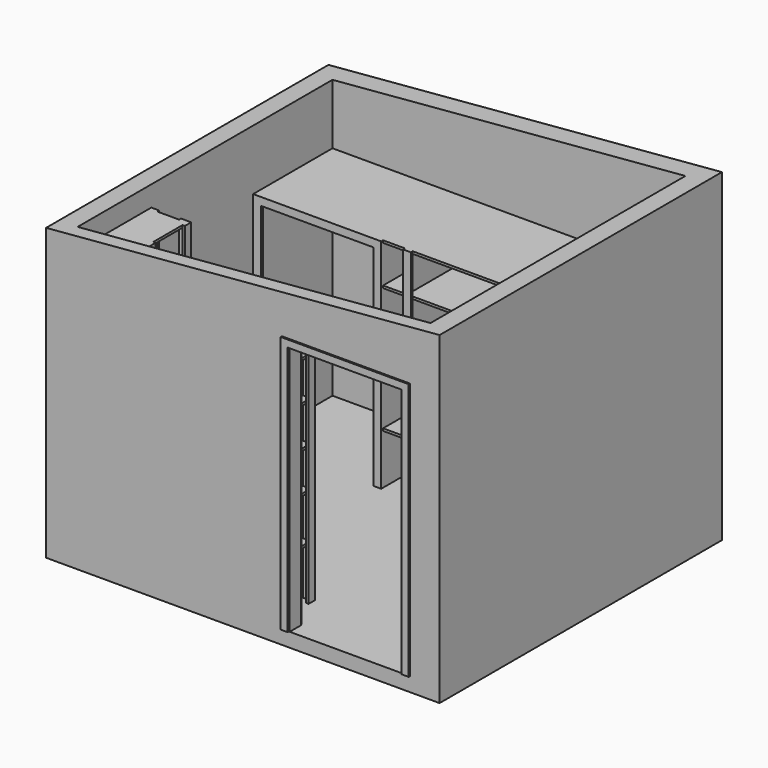
from build123d import *

# Parameters (mm, degrees)
F0_W      = 2590.8
F0_H      = 2520.95
F1_DEPTH  = 165.1
F2_W      = 3035.3
F2_H      = 2520.95
F3_DEPTH  = 114.3
F4_W      = 3035.3
F4_H      = 2520.95
F5_DEPTH  = 165.1
F6_W      = 2870.2
F6_H      = 2520.95
F7_DEPTH  = 165.1
F10_DEPTH = 2870.201
F8_W      = 914.4
F8_H      = 2032
F11_DEPTH = 114.3
F12_W     = 3200.4
F12_H     = 2870.2
F13_DEPTH = 114.3
F15_DEPTH = 12.7
F18_W     = 1651
F18_H     = 19.05
F19_DEPTH = 304.8
F20_W     = 1651
F20_H     = 38.1
F21_DEPTH = 19.05
F22_W     = 19.05
F22_H     = 63.5
F22_W_2   = 63.5
F22_H_2   = 19.05
F23_DEPTH = 2095.5
F24_W     = 2286
F24_H     = 19.05
F25_DEPTH = 304.8
F26_W     = 1422.4
F26_H     = 787.4
F26_W_2   = 990.6
F27_DEPTH = 990.6
F28_W     = 19.05
F28_H     = 787.4
F28_W_2   = 63.5
F28_H_2   = 19.05
F29_DEPTH = 1447.8
F30_W     = 19.05
F30_H     = 787.4
F31_DEPTH = 19.05
F32_W     = 2565.4
F32_H     = 787.4
F33_DEPTH = 19.05
F34_W     = 1631.95
F34_H     = 19.05
F35_DEPTH = 787.4
F36_W     = 1219.2
F36_H     = 2266.95
F37_DEPTH = 2520.951
F38_W     = 63.5
F38_H     = 19.05
F38_W_2   = 19.05
F38_H_2   = 787.4
F39_DEPTH = 1771.65
F40_W     = 19.05
F40_H     = 787.4
F41_DEPTH = 19.05
F42_W     = 2870.2
F42_H     = 787.4
F43_DEPTH = 19.05
F44_W     = 19.05
F44_H     = 323.85
F45_DEPTH = 787.4
F46_W     = 63.5
F46_H     = 19.05
F47_DEPTH = 323.85
F48_W     = 177.8
F48_H     = 19.05
F49_DEPTH = 787.4
F50_W     = 406.4
F50_H     = 19.05
F51_DEPTH = 304.8
F52_W     = 19.05
F52_H     = 63.5
F52_W_2   = 63.5
F52_H_2   = 19.05
F53_DEPTH = 2095.5
F54_W     = 914.4
F54_H     = 44.45
F54_H_2   = 19.05
F55_DEPTH = 19.05


# Not quite as in the source:
# - a pattern or mirror of a feature is missing from the dataset's text; its kind, count and spacing are read off the source's solid


with BuildPart() as f1:
    # F0 (on Right) → F1 (new body)
    with BuildSketch(Plane.YZ):
        with Locations((1295.4, 1260.475)):
            Rectangle(F0_W, F0_H)
    extrude(amount=F1_DEPTH)

    # F2 (on face) → F3 (join)
    with BuildSketch(Plane.XZ):
        with Locations((1517.65, 1260.475)):
            Rectangle(F2_W, F2_H)
    extrude(amount=F3_DEPTH)

    # F4 (on face) → F5 (join)
    with BuildSketch(Plane(origin=(0, 2590.8, 0), x_dir=(-1, 0, 0), z_dir=(0, 1, 0))):
        with Locations((-1517.65, 1260.475)):
            Rectangle(F4_W, F4_H)
    extrude(amount=F5_DEPTH)

    # F6 (on face) → F7 (join)
    with BuildSketch(Plane.YZ.offset(3035.3)):
        with Locations((1320.8, 1260.475)):
            Rectangle(F6_W, F6_H)
    extrude(amount=F7_DEPTH)

    # F9 (on face) → F10 (cut, through all)
    with BuildSketch(Plane.XZ.offset(114.3)):
        Polygon((0, 2520.95), (0, 2247.9), (3200.4, 2520.95), align=None)
    extrude(amount=-F10_DEPTH, mode=Mode.SUBTRACT)

    # F8 (on face) → F11 (cut)
    with BuildSketch(Plane.XZ.offset(114.3)):
        with Locations((2438.4, 1016)):
            Rectangle(F8_W, F8_H)
    extrude(amount=-F11_DEPTH, mode=Mode.SUBTRACT)

    # F12 (on face) → F13 (join)
    with BuildSketch(Plane(origin=(0, 0, 0), x_dir=(1, 0, 0), z_dir=(0, 0, -1))):
        with Locations((1600.2, -1320.8)):
            Rectangle(F12_W, F12_H)
    extrude(amount=F13_DEPTH)

    # F14 (on face) → F15 (join)
    with BuildSketch(Plane(origin=(0, 0, 0), x_dir=(-1, 0, 0), z_dir=(0, 1, 0))):
        Polygon((-1974.85, 2038.35), (-1974.85, 0), (-1917.7, 0), (-1917.7, 2095.5), (-2959.1, 2095.5), (-2959.1, 0), (-2901.95, 0), (-2901.95, 2038.35), align=None)
    f15 = extrude(amount=F15_DEPTH)

    # F15_copies: F15 across plane
    add(f15.mirror(Plane(origin=(0, -57.15, 0), x_dir=(0, 0, -1), z_dir=(0, -1, 0))))

    # F18 (on face) → F19 (join)
    with BuildSketch(Plane(origin=(0, 0, 0), x_dir=(-1, 0, 0), z_dir=(0, 1, 0))):
        with Locations((-990.6, 415.925)):
            Rectangle(F18_W, F18_H)
        with Locations((-990.6, 790.575)):
            Rectangle(F18_W, F18_H)
        with Locations((-990.6, 1114.425)):
            Rectangle(F18_W, F18_H)
        with Locations((-990.6, 1438.275)):
            Rectangle(F18_W, F18_H)
        with Locations((-990.6, 1762.125)):
            Rectangle(F18_W, F18_H)
        with Locations((-990.6, 2085.975)):
            Rectangle(F18_W, F18_H)
    extrude(amount=F19_DEPTH)

    # F20 (on face) → F21 (join)
    with BuildSketch(Plane(origin=(0, 0, 0), x_dir=(-1, 0, 0), z_dir=(0, 1, 0))):
        with Locations((-990.6, 2057.4)):
            Rectangle(F20_W, F20_H)
        with Locations((-990.6, 1733.55)):
            Rectangle(F20_W, F20_H)
        with Locations((-990.6, 1409.7)):
            Rectangle(F20_W, F20_H)
        with Locations((-990.6, 1085.85)):
            Rectangle(F20_W, F20_H)
        with Locations((-990.6, 387.35)):
            Rectangle(F20_W, F20_H)
        with Locations((-990.6, 762)):
            Rectangle(F20_W, F20_H)
    extrude(amount=F21_DEPTH)

    # F22 (on face) → F23 (join)
    with BuildSketch(Plane.XY):
        with Locations((1825.625, 31.75)):
            Rectangle(F22_W, F22_H)
        Polygon((1816.1, 260.35), (1835.15, 260.35), (1835.15, 323.85), (1816.1, 323.85), (1816.1, 304.8), align=None)
        with Locations((1784.35, 314.325)):
            Rectangle(F22_W_2, F22_H_2)
        with Locations((1358.9, 314.325)):
            Rectangle(F22_W_2, F22_H_2)
        Polygon((533.4, 304.8), (533.4, 323.85), (488.95, 323.85), (469.9, 323.85), (469.9, 304.8), align=None)
        with Locations((479.425, 355.6)):
            Rectangle(F22_W, F22_H)
        with Locations((927.1, 314.325)):
            Rectangle(F22_W_2, F22_H_2)
    extrude(amount=F23_DEPTH)

    # F24 (on face) → F25 (join)
    with BuildSketch(Plane.YZ.offset(165.1)):
        with Locations((1447.8, 2085.975)):
            Rectangle(F24_W, F24_H)
        with Locations((1447.8, 1762.125)):
            Rectangle(F24_W, F24_H)
        with Locations((1447.8, 1438.275)):
            Rectangle(F24_W, F24_H)
        with Locations((1447.8, 415.925)):
            Rectangle(F24_W, F24_H)
        with Locations((1447.8, 790.575)):
            Rectangle(F24_W, F24_H)
        with Locations((1447.8, 1114.425)):
            Rectangle(F24_W, F24_H)
    extrude(amount=F25_DEPTH)

    # F26 (on face) → F27 (cut)
    with BuildSketch(Plane.XY.offset(425.45)):
        with Locations((1333.5, 2197.1)):
            Rectangle(F26_W, F26_H)
        with Locations((2540, 2197.1)):
            Rectangle(F26_W_2, F26_H)
    extrude(amount=F27_DEPTH, mode=Mode.SUBTRACT)

    # F28 (on face) → F29 (join)
    with BuildSketch(Plane.XY):
        Polygon((1447.8, 1803.4), (1403.35, 1803.4), (1384.3, 1803.4), (1384.3, 1784.35), (1447.8, 1784.35), align=None)
        with Locations((1393.825, 2197.1)):
            Rectangle(F28_W, F28_H)
        with Locations((3003.55, 1793.875)):
            Rectangle(F28_W_2, F28_H_2)
    extrude(amount=F29_DEPTH)

    # F30 (on face) → F31 (cut)
    with BuildSketch(Plane.XY.offset(1447.8)):
        with Locations((1393.825, 2197.1)):
            Rectangle(F30_W, F30_H)
    extrude(amount=-F31_DEPTH, mode=Mode.SUBTRACT)

    # F32 (on face) → F33 (join)
    with BuildSketch(Plane.XY.offset(1428.75)):
        with Locations((1752.6, 2197.1)):
            Rectangle(F32_W, F32_H)
    extrude(amount=F33_DEPTH)

    # F34 (on face) → F35 (join)
    with BuildSketch(Plane.XZ.offset(-2590.8)):
        with Locations((2219.325, 415.925)):
            Rectangle(F34_W, F34_H)
    extrude(amount=F35_DEPTH)

    # F36 (on face) → F37 (cut, through all)
    with BuildSketch(Plane.XY):
        with Locations((774.7, 1457.325)):
            Rectangle(F36_W, F36_H)
    extrude(amount=F37_DEPTH, mode=Mode.SUBTRACT)

    # F38 (on face) → F39 (join)
    with BuildSketch(Plane.XY):
        with Locations((196.85, 1793.875)):
            Rectangle(F38_W, F38_H)
        with Locations((1196.975, 2197.1)):
            Rectangle(F38_W_2, F38_H_2)
        Polygon((1206.5, 1784.35), (1206.5, 1803.4), (1187.45, 1803.4), (1143, 1803.4), (1143, 1784.35), align=None)
    extrude(amount=F39_DEPTH)

    # F40 (on face) → F41 (cut)
    with BuildSketch(Plane.XY.offset(1771.65)):
        with Locations((1196.975, 2197.1)):
            Rectangle(F40_W, F40_H)
    extrude(amount=-F41_DEPTH, mode=Mode.SUBTRACT)

    # F42 (on face) → F43 (join)
    with BuildSketch(Plane.XY.offset(1752.6)):
        with Locations((1600.2, 2197.1)):
            Rectangle(F42_W, F42_H)
    extrude(amount=F43_DEPTH)

    # F44 (on face) → F45 (join)
    with BuildSketch(Plane.XZ.offset(-2590.8)):
        with Locations((1393.825, 1590.675)):
            Rectangle(F44_W, F44_H)
    extrude(amount=F45_DEPTH)

    # F46 (on face) → F47 (join, through all)
    with BuildSketch(Plane.XY.offset(1447.8)):
        with Locations((1416.05, 1793.875)):
            Rectangle(F46_W, F46_H)
        with Locations((3003.55, 1793.875)):
            Rectangle(F46_W, F46_H)
    extrude(amount=F47_DEPTH)

    # F48 (on face) → F49 (join)
    with BuildSketch(Plane.XZ.offset(-1803.4)):
        with Locations((1295.4, 415.925)):
            Rectangle(F48_W, F48_H)
        with Locations((1295.4, 790.575)):
            Rectangle(F48_W, F48_H)
        with Locations((1295.4, 1114.425)):
            Rectangle(F48_W, F48_H)
        with Locations((1295.4, 1438.275)):
            Rectangle(F48_W, F48_H)
    extrude(amount=-F49_DEPTH)

    # F50 (on face) → F51 (join)
    with BuildSketch(Plane.YZ.offset(165.1)):
        with Locations((527.05, 415.925)):
            Rectangle(F50_W, F50_H)
        with Locations((527.05, 790.575)):
            Rectangle(F50_W, F50_H)
        with Locations((527.05, 1114.425)):
            Rectangle(F50_W, F50_H)
        with Locations((527.05, 1438.275)):
            Rectangle(F50_W, F50_H)
        with Locations((527.05, 1762.125)):
            Rectangle(F50_W, F50_H)
        with Locations((527.05, 2085.975)):
            Rectangle(F50_W, F50_H)
    extrude(amount=F51_DEPTH)

    # F52 (on face) → F53 (join, through all)
    with BuildSketch(Plane.XY):
        with Locations((479.425, 355.6)):
            Rectangle(F52_W, F52_H)
        Polygon((469.9, 730.25), (469.9, 685.8), (488.95, 685.8), (488.95, 749.3), (469.9, 749.3), align=None)
        with Locations((438.15, 739.775)):
            Rectangle(F52_W_2, F52_H_2)
        with Locations((196.85, 739.775)):
            Rectangle(F52_W_2, F52_H_2)
    extrude(amount=F53_DEPTH)

    # F54 (on face) → F55 (join)
    with BuildSketch(Plane.XZ.offset(-1803.4)):
        with Locations((685.8, 1730.375)):
            Rectangle(F54_W, F54_H)
        with Locations((685.8, 1762.125)):
            Rectangle(F54_W, F54_H_2)
    extrude(amount=F55_DEPTH)


solid = f1.part
